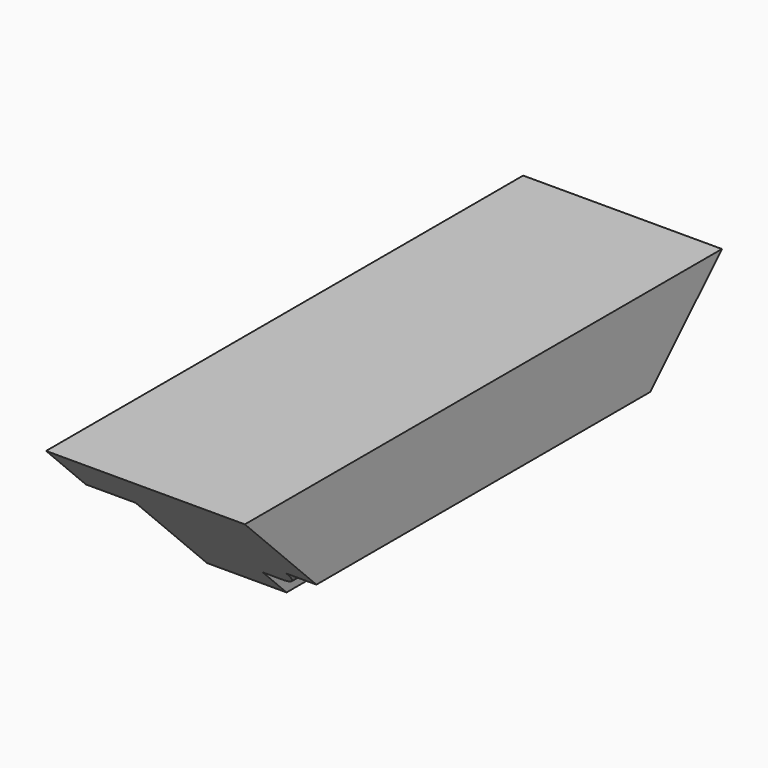
from build123d import *

# Parameters (mm, degrees)
F1_DEPTH = 152.4
F3_DEPTH = 50.8
F5_DEPTH = 50.8
F6_R     = 5.07999


# Not quite as in the source:
# - a fillet or chamfer is up to 0.001 mm smaller than in the source, because OpenCascade refuses the exact size


with BuildPart() as f1:
    # F0 (on Front) → F1 (new body)
    with BuildSketch(Plane.XZ):
        Polygon((25.4, 35.56), (-25.4, 35.56), (-25.4, 22.86), (-12.7, 22.86), (-12.7, 0), (0, 0), (7.62, 0), (7.62, 7.62), (17.78, 7.62), (17.78, 12.7), (25.4, 12.7), align=None)
    extrude(amount=F1_DEPTH)

    # F2 (on face) → F3 (cut)
    with BuildSketch(Plane.YZ.offset(25.4)):
        Polygon((-116.84, 0), (-152.4, 35.56), (-152.4, 0), align=None)
    extrude(amount=-F3_DEPTH, mode=Mode.SUBTRACT)

    # F4 (on face) → F5 (cut)
    with BuildSketch(Plane.YZ.offset(25.4)):
        Polygon((0, 0), (0, 35.56), (-35.56, 0), align=None)
    extrude(amount=-F5_DEPTH, mode=Mode.SUBTRACT)

    # F6 (radius 5.08 in the source; OpenCascade refuses exactly that, so slightly less here)
    f6_edges = [f1.edges().sort_by_distance(p)[0] for p in [
        (17.78, -76.2, 7.62),
    ]]
    fillet(f6_edges, radius=F6_R)


solid = f1.part
